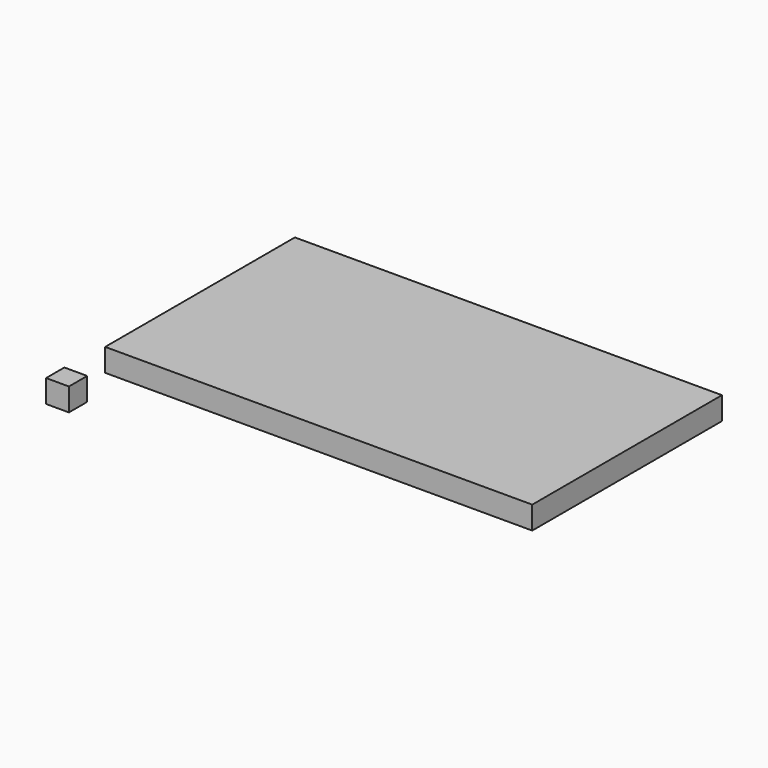
from build123d import *

# Parameters (mm, degrees)
F0_W     = 189.865
F0_H     = 105.41
F1_DEPTH = 10.16
F0_W_2   = 10.16
F0_H_2   = 10.16


# Not quite as in the source:
# - the program builds the solid bodies; features that only make, move or delete a surface that nothing else refers to are left out


with BuildPart() as f1:
    # F0 (on Top) → F1 (new body)
    with BuildSketch(Plane.XY):
        with Locations((-123.3860363317, 9.8514024484)):
            Rectangle(F0_W, F0_H)
    extrude(amount=F1_DEPTH)


with BuildPart() as f1b:
    # F0 (on Top) → F1, piece 2 (new body)
    with BuildSketch(Plane.XY):
        with Locations((-214.6248970795, -68.8832099867)):
            Rectangle(F0_W_2, F0_H_2)
    extrude(amount=F1_DEPTH)


solid = Compound([f1.part, f1b.part])
